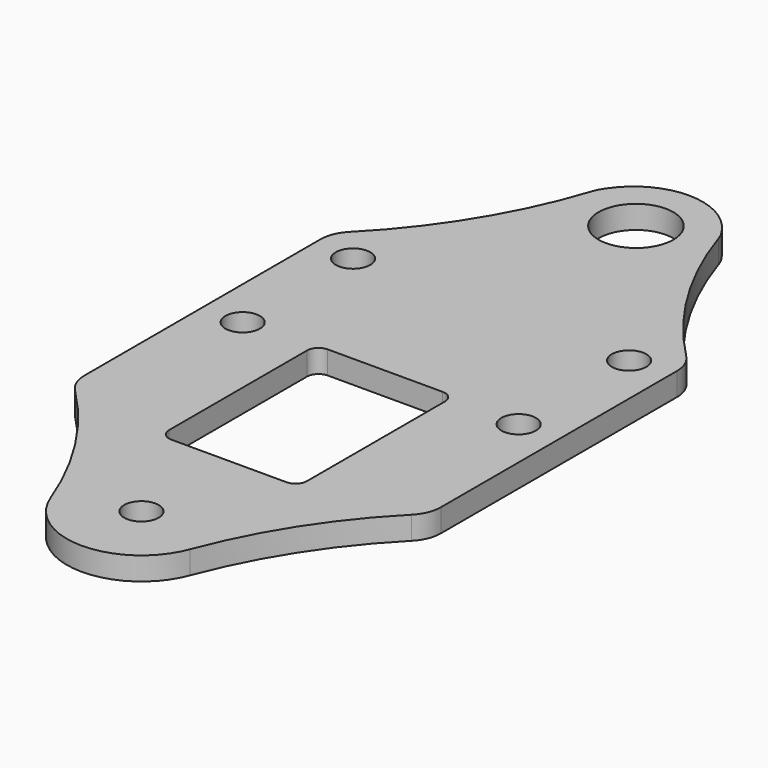
from build123d import *

# Parameters (mm, degrees)
F0_R     = 1.5
F0_R_2   = 3.25
F1_DEPTH = 2
F2_R     = 3
F3_W     = 12
F3_H     = 17
F4_DEPTH = 25
F5_R     = 1


with BuildPart() as f1:
    # F0 (on Top) → F1 (new body)
    with BuildSketch(Plane.XY):
        with BuildLine():
            Line((-15.5, 14.0758867192), (-15.5, -14.0758867192))
            ThreePointArc((-15.5, -14.0758867192), (-9.9776979071, -20.6460779619), (-6.0661514917, -28.2856485004))
            ThreePointArc((-6.0661514917, -28.2856485004), (0, -32.4824673534), (6.0661514917, -28.2856485004))
            ThreePointArc((6.0661514917, -28.2856485004), (9.9776979071, -20.6460779619), (15.5, -14.0758867192))
            Line((15.5, -14.0758867192), (15.5, 14.0758867192))
            ThreePointArc((15.5, 14.0758867192), (9.4126848848, 21.5229485882), (5.3843378024, 30.2571661019))
            Line((5.3843378024, 30.2571661019), (4.948926344, 30.8923631943))
            ThreePointArc((4.948926344, 30.8923631943), (0, 33.5), (-4.948926344, 30.8923631943))
            Line((-4.948926344, 30.8923631943), (-5.3843378024, 30.2571661019))
            ThreePointArc((-5.3843378024, 30.2571661019), (-9.4126848848, 21.5229485882), (-15.5, 14.0758867192))
        make_face()
        with Locations((0, -26)):
            Circle(F0_R, mode=Mode.SUBTRACT)
        with Locations((-12, 0)):
            Circle(F0_R, mode=Mode.SUBTRACT)
        with Locations((12, 0)):
            Circle(F0_R, mode=Mode.SUBTRACT)
        with Locations((-12, 12)):
            Circle(F0_R, mode=Mode.SUBTRACT)
        with Locations((0, 27.75)):
            Circle(F0_R_2, mode=Mode.SUBTRACT)
        with Locations((12, 12)):
            Circle(F0_R, mode=Mode.SUBTRACT)
    extrude(amount=F1_DEPTH)

    # F2
    f2_edges = [f1.edges().sort_by_distance(p)[0] for p in [
        (-15.5, 14.075887, 1),
        (5.384338, 30.257166, 1),
        (-5.384338, 30.257166, 1),
        (-15.5, -14.075887, 1),
        (15.5, -14.075887, 1),
        (15.5, 14.075887, 1),
    ]]
    fillet(f2_edges, radius=F2_R)

    # F3 (on face) → F4 (cut)
    with BuildSketch(Plane.XY.offset(2)):
        with Locations((0, -8)):
            Rectangle(F3_W, F3_H)
    extrude(amount=-F4_DEPTH, mode=Mode.SUBTRACT)

    # F5
    f5_edges = [f1.edges().sort_by_distance(p)[0] for p in [
        (-6, 0.5, 1),
        (6, 0.5, 1),
        (6, -16.5, 1),
        (-6, -16.5, 1),
    ]]
    fillet(f5_edges, radius=F5_R)


solid = f1.part
